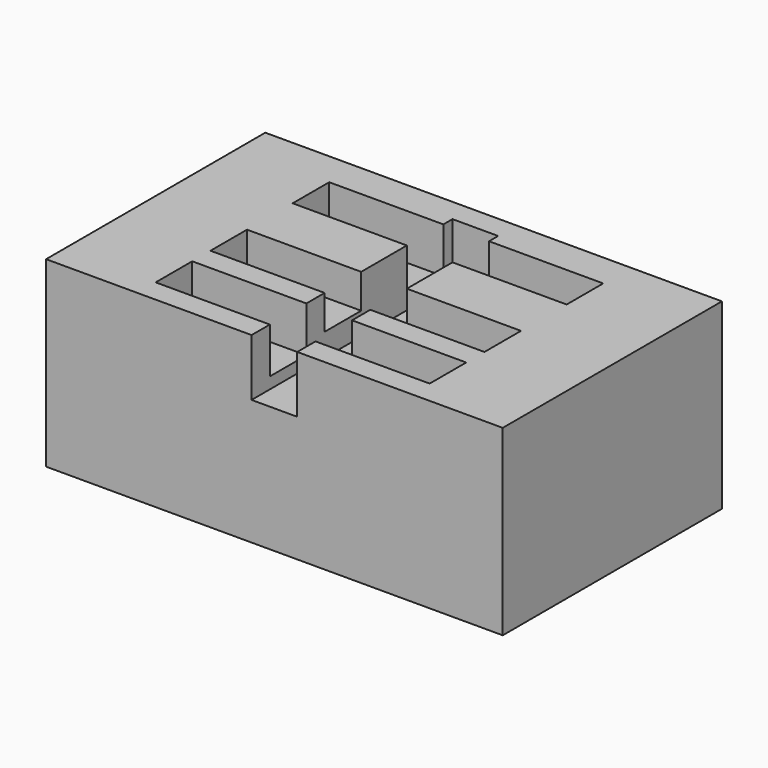
from build123d import *

# Parameters (mm, degrees)
F0_W     = 63.5
F0_H     = 38.1
F1_DEPTH = 25.4
F2_W     = 6.35
F2_H     = 34.925
F4_DEPTH = 7.9375
F3_W     = 15.875
F3_H     = 6.35
F5_DEPTH = 6.35
F6_DEPTH = 4.7625


# Not quite as in the source:
# - a length typed as a fraction of an inch, garbled in the dataset ("3 / 203.2 mm" for 3/8 in), is restored


with BuildPart() as f1:
    # F0 (on Top) → F1 (new body)
    with BuildSketch(Plane.XY):
        Rectangle(F0_W, F0_H)
    extrude(amount=F1_DEPTH)

    # F2 (on face) → F4 (cut)
    with BuildSketch(Plane.XY.offset(25.4)):
        with Locations((0, -1.5875)):
            Rectangle(F2_W, F2_H)
    extrude(amount=-F4_DEPTH, mode=Mode.SUBTRACT)

    # F3 (on face) → F5 (cut)
    with BuildSketch(Plane.XY.offset(25.4)):
        with Locations((11.1125, 11.1125)):
            Rectangle(F3_W, F3_H)
        with Locations((-11.1125, 11.1125)):
            Rectangle(F3_W, F3_H)
        with Locations((11.1125, -12.7)):
            Rectangle(F3_W, F3_H)
        with Locations((-11.1125, -12.7)):
            Rectangle(F3_W, F3_H)
    extrude(amount=-F5_DEPTH, mode=Mode.SUBTRACT)

    # F3 (on face) → F6 (cut)
    with BuildSketch(Plane.XY.offset(25.4)):
        with Locations((11.1125, -3.175)):
            Rectangle(F3_W, F3_H)
        with Locations((-11.1125, -3.175)):
            Rectangle(F3_W, F3_H)
    extrude(amount=-F6_DEPTH, mode=Mode.SUBTRACT)


solid = f1.part
